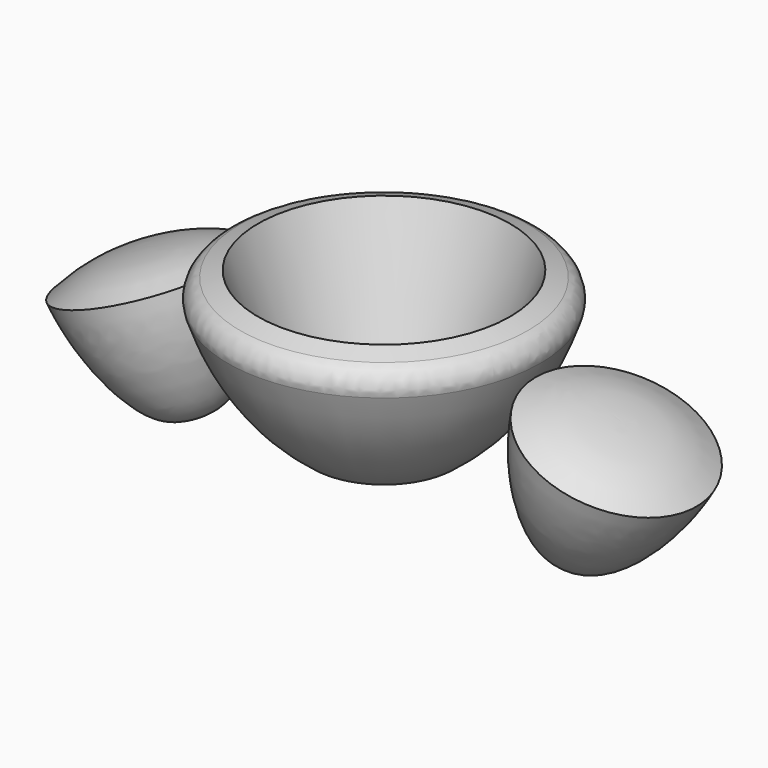
from build123d import *

# Parameters (mm, degrees)
F3_R = 2.65
F5_R = 0.4


# Not quite as in the source:
# - an extrude whose draft closes it to a point is written as a loft to that point


with BuildPart() as f1:
    # F0 (on Front) → F1 (revolve)
    with BuildSketch(Plane.XZ):
        with BuildLine():
            add(Edge.make_bspline(
                [(0, 13.816189227), (0.493117217, 13.816189227), (1.5042615966, 13.783137193), (2.6681258699, 13.4110701894), (3.2, 13.1832365588)],
                knots=[0, 0, 0, 0, 0.4783409697, 1, 1, 1, 1], degree=3))
            Line((0, 13.816189227), (0, 9.816189227))
            add(Edge.make_bspline(
                [(0, 9.816189227), (0.5371469513, 9.816189227), (2.2298259658, 10.7962754001), (3.0163129366, 12.4202263928), (3.2, 13.1832365588)],
                knots=[0, 0, 0, 0, 0.4802508239, 0.9716816175, 0.9716816175, 0.9716816175, 0.9716816175], degree=3))
        make_face()
    revolve(axis=Axis((0, 0, 11.816189227), (0, 0, -1)))

    # F3 (on offset) → F4 section 0
    with BuildSketch(Plane.XY.offset(13.85), mode=Mode.PRIVATE) as f4_s0:
        Circle(F3_R)
    loft([f4_s0.sketch, Vertex(0, 0, 6.5691848384)], ruled=True, mode=Mode.SUBTRACT)

    # F5
    f5_edges = [f1.edges().sort_by_distance(p)[0] for p in [
        (-3.2, 0, 13.183237),
    ]]
    fillet(f5_edges, radius=F5_R)


with BuildPart() as f7:
    # F6 (on Front) → F7 (revolve)
    with BuildSketch(Plane.XZ):
        with BuildLine():
            add(Edge.make_bspline(
                [(-3.0182146002, 12.5617515296), (-3.366192171, 12.601881569), (-3.9240989414, 12.5963100462), (-4.4119666474, 12.4530334641), (-4.7567621805, 12.3199066147)],
                knots=[0, 0, 0, 0, 0.5008877726, 1, 1, 1, 1], degree=3))
            Line((-4.7567621805, 12.3199066147), (-3.7385054336, 9.6826446378))
            add(Edge.make_bspline(
                [(-3.7385054336, 9.6826446378), (-3.3948102019, 9.8153466566), (-2.9667460836, 10.2097649857), (-2.8175992193, 11.6358339578), (-3.0182146002, 12.5617515296)],
                knots=[0, 0, 0, 0, 0.378560841, 1, 1, 1, 1], degree=3))
        make_face()
    revolve(axis=Axis((-2.3783810902, 0, 6.1599533074), (-0.36018832, 0, 0.9328796139)))


with BuildPart() as f8_1:
    # F8: instance of F7
    add(f7.part.mirror(Plane.YZ))


solid = Compound([f1.part, f7.part, f8_1.part])
